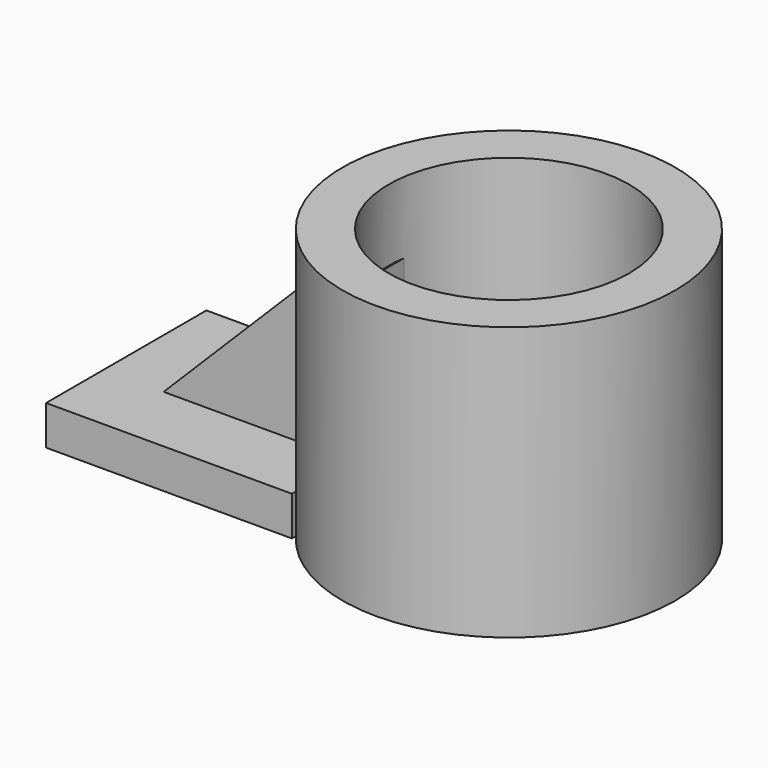
from build123d import *

# Parameters (mm, degrees)
F0_W        = 52.3398779333
F0_H        = 42.6720008254
F1_DEPTH    = 8.382
F2_R        = 35.438248993
F3_DEPTH    = 58.166
F4_R        = 25.617866598
F5_DEPTH    = 76.454
F6_W        = 48.6727505922
F6_H        = 15.6686254777
F7_DEPTH    = 42.926
F8_T4_DEPTH = 224.6950187396
F8_S5_R     = 35.438248993
F8_T6_DEPTH = 117


# Not quite as in the source:
# - a fillet or chamfer that OpenCascade refuses, or shapes differently, is made with other operations: its cross-section is extruded or revolved along the edge and cut away or added


with BuildPart() as f1:
    # F0 (on Top) → F1 (new body)
    with BuildSketch(Plane.XY):
        with Locations((-29.17031385, -1.0001249611)):
            Rectangle(F0_W, F0_H)
    extrude(amount=F1_DEPTH)

    # F2 (on Top) → F3 (join)
    with BuildSketch(Plane.XY):
        with Locations((25.3365002573, 0)):
            Circle(F2_R)
    extrude(amount=F3_DEPTH)

    # F4 (on Top) → F5 (cut)
    with BuildSketch(Plane.XY):
        with Locations((25.3365002573, 0)):
            Circle(F4_R)
    extrude(amount=F5_DEPTH, mode=Mode.SUBTRACT)

    # F6 (on Top) → F7 (join)
    with BuildSketch(Plane.XY):
        with Locations((-24.3363752961, 0.8334375452)):
            Rectangle(F6_W, F6_H)
    extrude(amount=F7_DEPTH)

    # F8: chamfer of 40.64 on 1 edges, made by hand


with BuildPart() as f8_tool2:
    # F8_s3 → F8_t4 (new body)
    with BuildSketch(Plane.XZ.offset(-113.180946915)):
        Polygon((-8.0327505922, 42.926), (-48.6727505922, 2.286), (-48.6727505922, 42.926), align=None)
    extrude(amount=F8_T4_DEPTH)

    # F8_s5 → F8_t6 (cut, symmetric)
    with BuildSketch(Plane.XY.offset(22.6)):
        with Locations((25.3365002573, 0)):
            Circle(F8_S5_R)
    extrude(amount=F8_T6_DEPTH, both=True, mode=Mode.SUBTRACT)

    split(bisect_by=Plane.XY.offset(8.382), keep=Keep.TOP)


with BuildPart() as f1_1:
    add(f1.part)

    # F8_t1: cut F8_tool2
    add(f8_tool2.part, mode=Mode.SUBTRACT)


solid = f1_1.part
